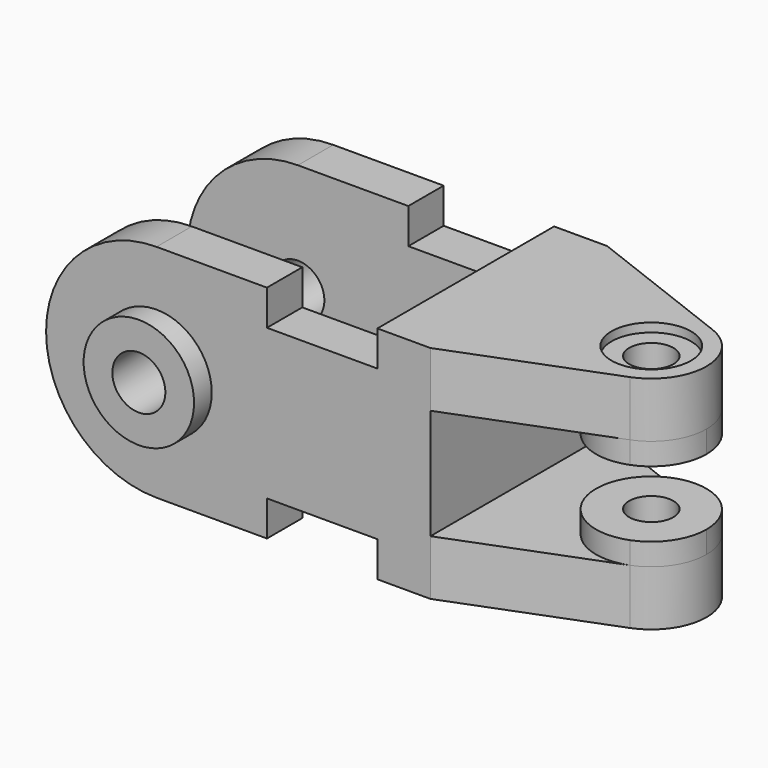
from build123d import *

# Parameters (mm, degrees)
F1_DEPTH        = 50
F2_W            = 25
F2_H            = 30
F3_DEPTH        = 50.001
F5_DEPTH        = 50
F6_W            = 42.5
F6_H            = 25
F7_DEPTH        = 50.001
F8_R            = 12.5
F9_DEPTH        = 5
F10_R           = 12.5
F11_DEPTH       = 5
F12_R           = 6
F13_DEPTH       = 201
F15_D           = 12
F17_DEPTH       = 5
F19_DEPTH       = 5
F21_D           = 10
F21_DEPTH       = 17.5
F21_CBORE_D     = 18
F21_CBORE_DEPTH = 2
F21_TIP         = 3.0043030951
F23_D           = 10
F23_DEPTH       = 17.5
F23_CBORE_D     = 18
F23_CBORE_DEPTH = 2
F23_TIP         = 3.0043030951


# Not quite as in the source:
# - an extrude ends at something that could not be found from the text; its depth is read off the source's solid


with BuildPart() as f1:
    # F0 (on Front) → F1 (new body)
    with BuildSketch(Plane.XZ):
        with BuildLine():
            Line((25, 25), (0, 25))
            ThreePointArc((0, 25), (-25, 0), (0, -25))
            Line((0, -25), (25, -25))
            Line((25, -25), (25, -17))
            Line((25, -17), (50, -17))
            Line((50, -17), (50, -25))
            Line((50, -25), (62, -25))
            Line((62, -25), (62, 0))
            Line((62, 0), (62, 25))
            Line((62, 25), (50, 25))
            Line((50, 25), (50, 17))
            Line((50, 17), (25, 17))
            Line((25, 17), (25, 25))
        make_face()
    extrude(amount=F1_DEPTH)

    # F2 (on face) → F3 (cut, through all)
    with BuildSketch(Plane.XY.offset(25)):
        with Locations((-12.5, -25)):
            Rectangle(F2_W, F2_H)
        with Locations((12.5, -25)):
            Rectangle(F2_W, F2_H)
        with Locations((37.5, -25)):
            Rectangle(F2_W, F2_H)
    extrude(amount=-F3_DEPTH, mode=Mode.SUBTRACT)

    # F4 (on face) → F5 (join)
    with BuildSketch(Plane.XY.offset(25)):
        with BuildLine():
            Line((62, -50), (96.5075043991, -36.6590052789))
            ThreePointArc((96.5075043991, -36.6590052789), (104.5, -25), (96.5075043991, -13.3409947211))
            Line((96.5075043991, -13.3409947211), (62, 0))
            Line((62, 0), (62, -50))
        make_face()
    extrude(amount=-F5_DEPTH)

    # F6 (on face) → F7 (cut, through all)
    with BuildSketch(Plane.XZ.offset(50)):
        with Locations((83.25, 0)):
            Rectangle(F6_W, F6_H)
    extrude(amount=-F7_DEPTH, mode=Mode.SUBTRACT)

    # F8 (on face) → F9 (join)
    with BuildSketch(Plane.XZ.offset(50)):
        Circle(F8_R)
    extrude(amount=F9_DEPTH)

    # F10 (on face) → F11 (join)
    with BuildSketch(Plane(origin=(0, 0, 0), x_dir=(-1, 0, 0), z_dir=(0, 1, 0))):
        Circle(F10_R)
    extrude(amount=F11_DEPTH)

    # F12 (on face) → F13 (cut, through all)
    with BuildSketch(Plane(origin=(0, 5, 0), x_dir=(-1, 0, 0), z_dir=(0, 1, 0))):
        Circle(F12_R)
    extrude(amount=F13_DEPTH, mode=Mode.SUBTRACT)

    # F15 (through all)
    with Locations(Plane.XZ.offset(55)):
        with Locations((0, 0)):
            Hole(F15_D / 2)

    # F16 (on face) → F17 (join)
    with BuildSketch(Plane.XY.offset(-12.5)):
        with BuildLine():
            ThreePointArc((96.5075043991, -36.6590052789), (102.3100389182, -32.0677505266), (104.5, -25))
            ThreePointArc((104.5, -25), (102.3100389182, -17.9322494734), (96.5075043991, -13.3409947211))
            ThreePointArc((96.5075043991, -13.3409947211), (79.5, -25), (96.5075043991, -36.6590052789))
        make_face()
    extrude(amount=F17_DEPTH)

    # F18 (on face) → F19 (join)
    with BuildSketch(Plane(origin=(0, 0, 12.5), x_dir=(1, 0, 0), z_dir=(0, 0, -1))):
        with BuildLine():
            ThreePointArc((96.5075043991, 13.3409947211), (102.3100389182, 17.9322494734), (104.5, 25))
            ThreePointArc((104.5, 25), (102.3100389182, 32.0677505266), (96.5075043991, 36.6590052789))
            ThreePointArc((96.5075043991, 36.6590052789), (79.5, 25), (96.5075043991, 13.3409947211))
        make_face()
    extrude(amount=F19_DEPTH)

    # F21
    with Locations(Plane.XY.offset(25)):
        with Locations((92, -25)):
            CounterBoreHole(F21_D / 2, F21_CBORE_D / 2, F21_CBORE_DEPTH, depth=F21_DEPTH)
            with Locations((0, 0, -(F21_DEPTH + F21_TIP / 2))):  # 118° drill point
                Cone(0, F21_D / 2, F21_TIP, mode=Mode.SUBTRACT)

    # F23
    with Locations(Plane(origin=(0, 0, -25), x_dir=(1, 0, 0), z_dir=(0, 0, -1))):
        with Locations((92, 25)):
            CounterBoreHole(F23_D / 2, F23_CBORE_D / 2, F23_CBORE_DEPTH, depth=F23_DEPTH)
            with Locations((0, 0, -(F23_DEPTH + F23_TIP / 2))):  # 118° drill point
                Cone(0, F23_D / 2, F23_TIP, mode=Mode.SUBTRACT)


solid = f1.part
